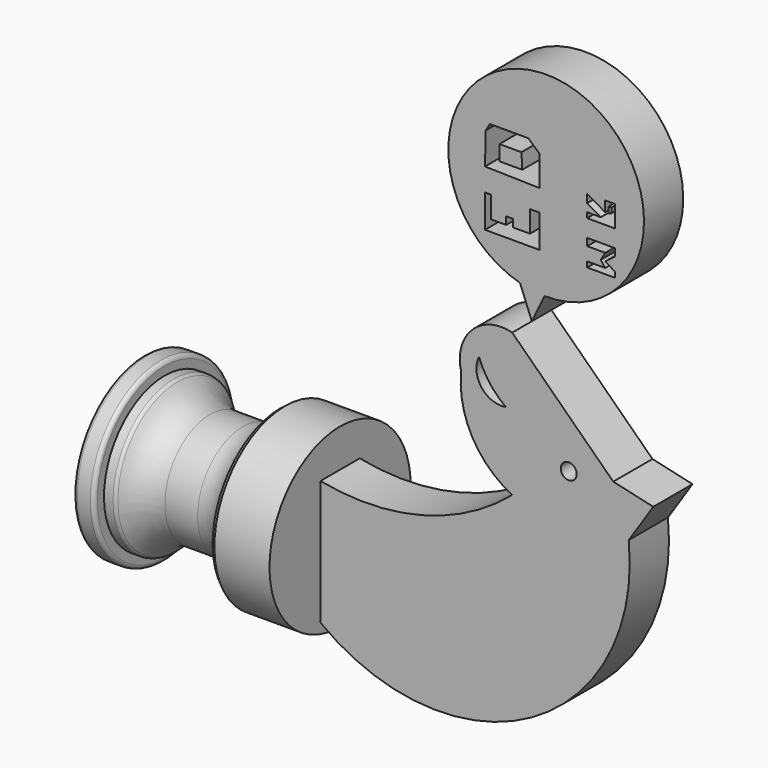
from build123d import *

# Parameters (mm, degrees)
F4_R      = 0.508
F7_DEPTH  = 3.175
F9_D      = 2.0574
F11_DEPTH = 12.7
F13_DEPTH = 3.175
F15_DEPTH = 12.7


# Not quite as in the source:
# - a fillet or chamfer that OpenCascade refuses, or shapes differently, is made with other operations: its cross-section is extruded or revolved along the edge and cut away or added


with BuildPart() as f1:
    # F0 (on Front) → F1 (revolve)
    with BuildSketch(Plane.XZ):
        Polygon((-25.4, 0), (0, 0), (0, 11.43), (-7.62, 11.43), (-7.62, 7.3114731075), (-20.32, 7.3114731075), (-21.2499899719, 9.835730216), (-22.7114037935, 9.835730216), (-22.7114037935, 11.43), (-25.4, 11.43), align=None)
    revolve(axis=Axis((-12.7, 0, 0), (-1, 0, 0)))

    # F2: fillet of radius 5.08 on 1 edges, made by hand

    # F2_s1 → F2_t2 (revolve)
    with BuildSketch(Plane.XZ):
        with BuildLine():
            ThreePointArc((-16.8597077176, 7.3114731075), (-19.3918240371, 7.9875218198), (-21.2499899719, 9.835730216))
            Line((-21.2499899719, 9.835730216), (-20.32, 7.3114731075))
            Line((-20.32, 7.3114731075), (-16.8597077176, 7.3114731075))
        make_face()
    revolve(axis=Axis((-20.32, 0, 0), (-1, 0, 0)))

    # F3: fillet of radius 5.08 on 1 edges, made by hand

    # F3_s1 → F3_t2 (revolve)
    with BuildSketch(Plane.XZ):
        with BuildLine():
            ThreePointArc((-7.62, 11.43), (-9.3738270483, 8.4741600369), (-12.6081829822, 7.3114731075))
            Line((-12.6081829822, 7.3114731075), (-7.62, 7.3114731075))
            Line((-7.62, 7.3114731075), (-7.62, 11.43))
        make_face()
    revolve(axis=Axis((-7.62, 0, 0), (-1, 0, 0)))

    # F4
    f4_edges = [f1.edges().sort_by_distance(p)[0] for p in [
        (-21.24999, 0, -9.83573),
        (-22.711404, 0, -11.43),
        (-25.4, 0, -11.43),
    ]]
    fillet(f4_edges, radius=F4_R)

    # F5: chamfer of 0.508 on 1 edges, made by hand

    # F5_s1 → F5_t2 (revolve, cut)
    with BuildSketch(Plane.XZ):
        with BuildLine():
            Line((-7.7429817287, 10.9728511125), (-7.1192910196, 11.442218632))
            Line((-7.1192910196, 11.442218632), (-7.1192910196, 11.452378632))
            ThreePointArc((-7.1192910196, 11.452378632), (-7.3696455098, 11.44016), (-7.62, 11.44016))
            Line((-7.62, 11.44016), (-7.629976366, 11.4319229462))
            ThreePointArc((-7.629976366, 11.4319229462), (-7.6800748035, 11.2010835053), (-7.7527446032, 10.9756639192))
            Line((-7.7527446032, 10.9756639192), (-7.7429817287, 10.9728511125))
        make_face()
    revolve(axis=Axis((-7.62, 0, 0), (-1, 0, 0)), mode=Mode.SUBTRACT)

    # F6 (on Front) → F7 (join, symmetric)
    with BuildSketch(Plane.XZ):
        with BuildLine():
            Line((0, 6.4907935448), (0, -9.6620609984))
            ThreePointArc((0, -9.6620609984), (27.3235808445, -11.5905018684), (39.9187803268, 12.7335172147))
            Line((39.9187803268, 12.7335172147), (43.1029349566, 17.5670832396))
            Line((43.1029349566, 17.5670832396), (37.9153452814, 18.7469273806))
            Line((37.9153452814, 18.7469273806), (24.8299874365, 31.4825810492))
            ThreePointArc((24.8299874365, 31.4825810492), (19.6194729327, 30.0910701799), (18.2263422757, 24.8809885234))
            ThreePointArc((18.2263422757, 24.8809885234), (19.6474301741, 17.8834645614), (24.8299874365, 12.9716489464))
            ThreePointArc((24.8299874365, 12.9716489464), (13.1623202589, 6.8680022006), (0, 6.4907935448))
        make_face()
    extrude(amount=F7_DEPTH, both=True)

    # F9 (through all)
    with Locations(Plane(origin=(0, 3.175, 0), x_dir=(-1, 0, 0), z_dir=(0, 1, 0))):
        with Locations((-32.1498028934, 18.0507935584)):
            Hole(F9_D / 2)

    # F10 (on face) → F11 (cut, symmetric)
    with BuildSketch(Plane(origin=(0, 3.175, 0), x_dir=(-1, 0, 0), z_dir=(0, 1, 0))):
        with BuildLine():
            ThreePointArc((-20.5308888108, 27.3354519159), (-21.9193644523, 24.7679811752), (-24.0082591772, 22.7292831987))
            ThreePointArc((-24.0082591772, 22.7292831987), (-20.8428543324, 23.9552831131), (-20.5308888108, 27.3354519159))
        make_face()
    extrude(amount=F11_DEPTH, both=True, mode=Mode.SUBTRACT)


with BuildPart() as f13:
    # F12 (on face) → F13 (new body, symmetric)
    with BuildSketch(Plane(origin=(0, 3.175, 0), x_dir=(-1, 0, 0), z_dir=(0, 1, 0))):
        with BuildLine():
            Line((-26.4666415751, 34.8943322897), (-24.8299874365, 31.4825810492))
            Line((-24.8299874365, 31.4825810492), (-23.3040340245, 35.3521183133))
            ThreePointArc((-23.3040340245, 35.3521183133), (-28.5012203621, 60.1034931642), (-26.4666415751, 34.8943322897))
        make_face()
    extrude(amount=F13_DEPTH, both=True)

    # F14 (on face) → F15 (cut, symmetric)
    with BuildSketch(Plane(origin=(0, 6.35, 0), x_dir=(-1, 0, 0), z_dir=(0, 1, 0))):
        Polygon((-35.6027372181, 39.9427898228), (-31.9911800325, 39.9427898228), (-31.9911800325, 40.6517386436), (-34.3299508095, 40.6517386436), (-33.757902766, 41.3867458701), (-34.3299508095, 42.3773415387), (-31.9911800325, 42.3773415387), (-31.9911800325, 43.3226935565), (-35.6027372181, 43.3226935565), (-35.6027372181, 42.3773415387), (-34.3299508095, 41.3867458701), (-35.6027372181, 40.6517386436), align=None)
        Polygon((-35.6027372181, 45.567497611), (-31.9911800325, 45.567497611), (-31.9911800325, 46.2499822183), (-33.757902766, 46.2499822183), (-31.9911800325, 47.2702272236), (-31.9911800325, 48.3551248908), (-34.3299508095, 47.0000132918), (-34.3299508095, 48.3551248908), (-35.6027372181, 48.3551248908), align=None)
        Polygon((-34.7663201392, 47.0000132918), (-35.1461172104, 47.1575073898), (-35.1461172104, 47.8113219142), (-34.7663201392, 47.8113219142), align=None, mode=Mode.SUBTRACT)
        Polygon((-25.8445478976, 44.1996492445), (-25.8445478976, 39.9427898228), (-18.765181303, 39.9427898228), (-18.765181303, 44.1996492445), (-19.5589084178, 44.1996492445), (-19.5589084178, 41.3867458701), (-21.5028319508, 41.3867458701), (-21.5028319508, 42.3773415387), (-22.3683007061, 42.3773415387), (-22.3683007061, 41.3867458701), (-24.5892498642, 41.3867458701), (-24.5892498642, 44.1996492445), align=None)
        Polygon((-25.8445478976, 50.8860163391), (-25.8445478976, 47.0000132918), (-18.765181303, 47.1575073898), (-18.8570892325, 51.2887728417), (-19.388453251, 52.2089174014), (-24.377239868, 52.2089174014), align=None)
        Polygon((-20.6333789974, 48.3551248908), (-23.5887039453, 48.3551248908), (-23.4892610461, 50.3255613148), (-20.6333789974, 50.3255613148), align=None, mode=Mode.SUBTRACT)
    extrude(amount=F15_DEPTH, both=True, mode=Mode.SUBTRACT)


solid = Compound([f1.part, f13.part])
